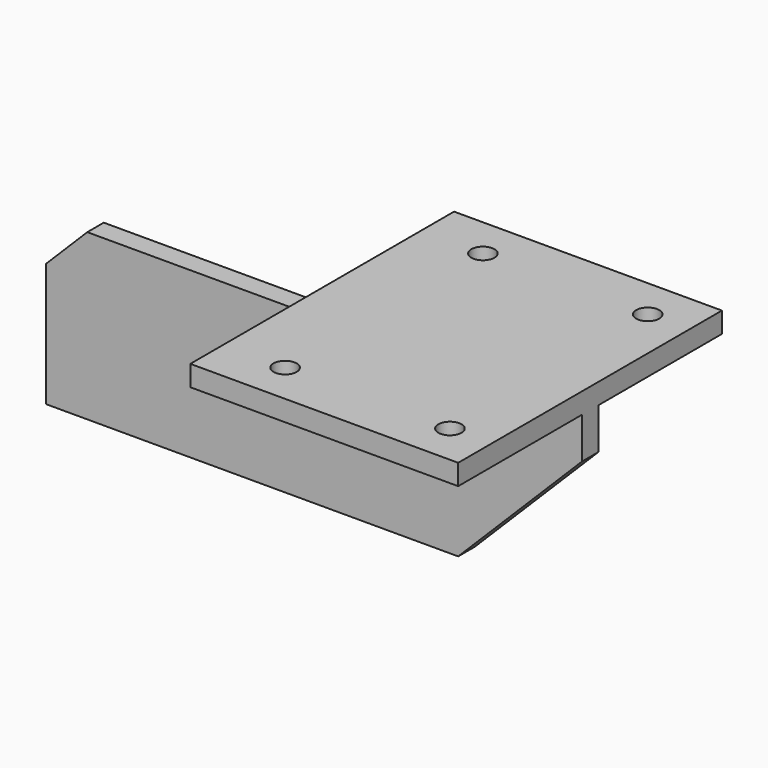
from build123d import *

# Parameters (mm, degrees)
F0_W     = 165.1
F0_H     = 203.2
F1_DEPTH = 12.7
F3_D     = 14.2875
F3_DEPTH = 50.8
F3_TIP   = 4.2923980472
F4_W     = 330.2
F4_H     = 12.7
F5_DEPTH = 101.6
F6_SIZE  = 76.2
F7_SIZE  = 25.4


# Not quite as in the source:
# - a length typed as a fraction of an inch, garbled in the dataset ("3 / 203.2 mm" for 3/8 in), is restored


with BuildPart() as f1:
    # F0 (on Top) → F1 (new body)
    with BuildSketch(Plane.XY):
        Rectangle(F0_W, F0_H)
    extrude(amount=F1_DEPTH)

    # F3
    with Locations(Plane.XY.offset(12.7)):
        with Locations((-44.45, 76.2), (57.15, 76.2), (-44.45, -76.2), (57.15, -76.2)):
            Hole(F3_D / 2, depth=F3_DEPTH)
            with Locations((0, 0, -(F3_DEPTH + F3_TIP / 2))):  # 118° drill point
                Cone(0, F3_D / 2, F3_TIP, mode=Mode.SUBTRACT)

    # F4 (on face) → F5 (join)
    with BuildSketch(Plane(origin=(0, 0, 0), x_dir=(1, 0, 0), z_dir=(0, 0, -1))):
        with Locations((-82.55, 0)):
            Rectangle(F4_W, F4_H)
    extrude(amount=F5_DEPTH)

    # F6
    f6_edges = [f1.edges().sort_by_distance(p)[0] for p in [
        (82.55, 0, -101.6),
    ]]
    chamfer(f6_edges, length=F6_SIZE)

    # F7
    f7_edges = [f1.edges().sort_by_distance(p)[0] for p in [
        (-247.65, 0, 0),
    ]]
    chamfer(f7_edges, length=F7_SIZE)


solid = f1.part
